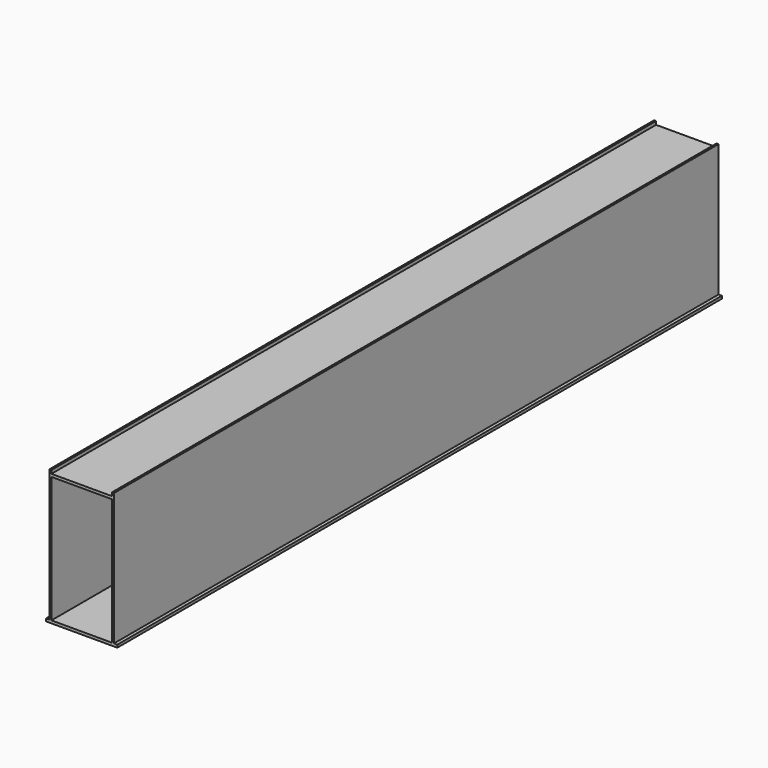
from build123d import *

# Parameters (mm, degrees)
F0_W     = 1143
F0_H     = 50.8
F1_DEPTH = 14285.9125


# Not quite as in the source:
# - a feature of the source that left no trace in its solid (it failed there, or was rolled back) is left out


with BuildPart() as f1:
    # F0 (on Front) → F1 (new body)
    with BuildSketch(Plane.XZ):
        Polygon((-636.190625, -1271.5875), (710.009375, -1271.5875), (710.009375, -1220.7875), (646.509375, -1220.7875), (608.409375, -1220.7875), (-534.590625, -1220.7875), (-572.690625, -1220.7875), (-636.190625, -1220.7875), align=None)
        Polygon((608.409375, -1220.7875), (646.509375, -1220.7875), (646.509375, 1281.1125), (608.409375, 1281.1125), (608.409375, 1217.6125), (608.409375, 1166.8125), align=None)
        Polygon((-572.690625, 1281.1125), (-572.690625, -1220.7875), (-534.590625, -1220.7875), (-534.590625, 1166.8125), (-534.590625, 1217.6125), (-534.590625, 1281.1125), align=None)
        with Locations((36.909375, 1192.2125)):
            Rectangle(F0_W, F0_H)
    extrude(amount=F1_DEPTH)


solid = f1.part
